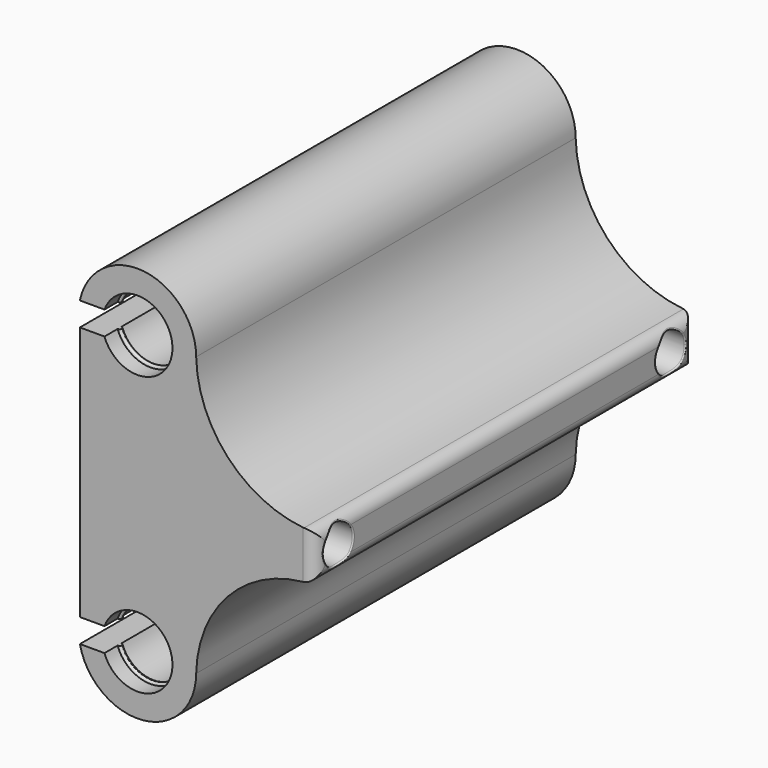
from build123d import *

# Parameters (mm, degrees)
F1_DEPTH      = 50.8
F2_R          = 4
F3_DEPTH      = 25.4
F4_T1_DEPTH   = 22.7
F4_T3_DEPTH   = 113.7216584723
F4_T5_DEPTH   = 113.721658441
F5_R          = 0.254
F8_DEPTH      = 0.9906
F11_T2_ANGLE  = 338.3178112703
F11_T4_ANGLE  = 338.3178112703
F11_T6_ANGLE  = 338.3178112703
F11_T8_ANGLE  = 338.3178112703
F11_T10_ANGLE = 338.3178112703
F11_T12_ANGLE = 338.3178112703
F11_T14_ANGLE = 338.3178112703
F11_T16_ANGLE = 338.3178112703


# Not quite as in the source:
# - a fillet or chamfer that OpenCascade refuses, or shapes differently, is made with other operations: its cross-section is extruded or revolved along the edge and cut away or added
# - ends of sketch curves that miss each other by under 0.0002 mm in the source are joined


with BuildPart() as f1:
    # F0 (on Front) → F1 (new body, symmetric)
    with BuildSketch(Plane.XZ):
        with BuildLine():
            ThreePointArc((-7.0574570763, 32.385), (7.50062, 29.845), (-7.0574570763, 27.305))
            Line((-7.0574570763, 27.305), (-12.3215420944, 27.305))
            Line((-12.3215420944, 27.305), (-12.3215420944, -27.305))
            Line((-12.3215420944, -27.305), (-7.0574570763, -27.305))
            ThreePointArc((-7.0574570763, -27.305), (7.50062, -29.845), (-7.0574570763, -32.385))
            Line((-7.0574570763, -32.385), (-12.3215420944, -32.385))
            ThreePointArc((-12.3215420944, -32.385), (1.2765893389, -42.3606829316), (12.58062, -29.845))
            ThreePointArc((12.58062, -29.845), (20.2152455374, -12.2439740194), (37.98062, -5))
            Line((37.98062, -5), (37.98062, 0))
            Line((37.98062, 0), (37.98062, 5))
            ThreePointArc((37.98062, 5), (20.2152461882, 12.2439733419), (12.58062, 29.845))
            ThreePointArc((12.58062, 29.845), (1.2765893389, 42.3606829316), (-12.3215420944, 32.385))
            Line((-12.3215420944, 32.385), (-7.0574570763, 32.385))
        make_face()
    extrude(amount=F1_DEPTH, both=True)

    # F2 (on face) → F3 (cut)
    with BuildSketch(Plane.YZ.offset(37.98062)):
        with Locations((-44.45, 0)):
            Circle(F2_R)
        with Locations((44.45, 0)):
            Circle(F2_R)
    extrude(amount=-F3_DEPTH, mode=Mode.SUBTRACT)

    # F4: fillet of radius 2.54 on 4 edges, made by hand

    # F4_s2 → F4_t1 (cut)
    with BuildSketch(Plane.XY.offset(-11.35)):
        with BuildLine():
            ThreePointArc((35.44062, -50.8), (37.2366712242, -50.0560512242), (37.98062, -48.26))
            Line((37.98062, -48.26), (37.98062, -50.8))
            Line((37.98062, -50.8), (35.44062, -50.8))
        make_face()
        with BuildLine():
            ThreePointArc((35.44062, 50.8), (37.2366712242, 50.0560512242), (37.98062, 48.26))
            Line((37.98062, 48.26), (37.98062, 50.8))
            Line((37.98062, 50.8), (35.44062, 50.8))
        make_face()
    extrude(amount=F4_T1_DEPTH, mode=Mode.SUBTRACT)

    # F4_s4 → F4_t3 (cut)
    with BuildSketch(Plane.XZ.offset(-56.8608292361)):
        with BuildLine():
            ThreePointArc((35.671477868, 5.1051553375), (37.3165169834, 4.2881549501), (37.98062, 2.5756683055))
            Line((37.98062, 2.5756683055), (37.98062, 5))
            ThreePointArc((37.98062, 5), (36.8248523945, 5.0263024486), (35.671477868, 5.1051553375))
        make_face()
    extrude(amount=F4_T3_DEPTH, mode=Mode.SUBTRACT)

    # F4_s6 → F4_t5 (cut)
    with BuildSketch(Plane.XZ.offset(-56.8608292205)):
        with BuildLine():
            ThreePointArc((35.6714778739, -5.1051553432), (37.3165169854, -4.2881549541), (37.98062, -2.5756683118))
            Line((37.98062, -2.5756683118), (37.98062, -5))
            ThreePointArc((37.98062, -5), (36.8248523974, -5.0263024516), (35.6714778739, -5.1051553432))
        make_face()
    extrude(amount=F4_T5_DEPTH, mode=Mode.SUBTRACT)

    # F5
    f5_edges = [f1.edges().sort_by_distance(p)[0] for p in [
        (37.543684, -44.45, 4),
        (37.98062, -47.951606, -1.933586),
        (37.98062, -40.69224, 1.370853),
        (37.98062, -47.951606, 1.933586),
        (37.98062, -40.69224, -1.370853),
        (37.973504, -48.45, 0),
        (37.543684, -44.45, -4),
        (37.543684, 44.45, 4),
        (37.97661, 48.402676, -0.613478),
        (37.97661, 48.402676, 0.613478),
        (37.543688, 44.44316, -3.999994),
        (37.98062, 47.951606, -1.933586),
        (37.98062, 47.951606, 1.933586),
        (37.98062, 40.45, 0),
    ]]
    fillet(f5_edges, radius=F5_R)

    # F7 (on offset) → F8 (join)
    with BuildSketch(Plane.XZ.offset(47.29988)):
        with BuildLine():
            ThreePointArc((-6.5149930518, 32.385), (6.99262, 29.845), (-6.5149930518, 27.305))
            Line((-6.5149930518, 27.305), (-7.0574570763, 27.305))
            ThreePointArc((-7.0574570763, 27.305), (7.50062, 29.845), (-7.0574570763, 32.385))
            Line((-7.0574570763, 32.385), (-6.5149930518, 32.385))
        make_face()
    extrude(amount=-F8_DEPTH)


with BuildPart() as f9_1:
    # F9: instance of F1
    add(f1.part.mirror(Plane.XY))


with BuildPart() as f1_1:
    add(f1.part)

    add(f9_1.part)  # F10 merges F9_1
    # F10: F9_1, F1 across plane
    add(f9_1.part.mirror(Plane.XZ))
    add(f1.part.mirror(Plane.XZ))

    # F11: fillet of radius 0.508 on 8 edges, made by hand

    # F11_s1 → F11_t2 (revolve, cut)
    with BuildSketch(Plane(origin=(5.5132355773, 0, 28.7891953424), x_dir=(0, 1, 0), z_dir=(-0.1880857941, 0, -0.9821526022))):
        with BuildLine():
            ThreePointArc((-47.29988, -13.1140405264), (-47.1510902448, -12.7548302815), (-46.79188, -12.6060405264))
            Line((-46.79188, -12.6060405264), (-47.29988, -12.6060405264))
            Line((-47.29988, -12.6060405264), (-47.29988, -13.1140405264))
        make_face()
    revolve(axis=Axis((0, -47.29988, 29.845), (0, 1, 0)), revolution_arc=F11_T2_ANGLE, mode=Mode.SUBTRACT)

    # F11_s3 → F11_t4 (revolve, cut)
    with BuildSketch(Plane(origin=(5.5132355773, 0, 28.7891953424), x_dir=(0, 1, 0), z_dir=(-0.1880857941, 0, -0.9821526022))):
        with BuildLine():
            ThreePointArc((-46.81728, -12.6060405264), (-46.4580697552, -12.7548302815), (-46.30928, -13.1140405264))
            Line((-46.30928, -13.1140405264), (-46.30928, -12.6060405264))
            Line((-46.30928, -12.6060405264), (-46.81728, -12.6060405264))
        make_face()
    revolve(axis=Axis((0, -46.30928, 29.845), (0, 1, 0)), revolution_arc=F11_T4_ANGLE, mode=Mode.SUBTRACT)

    # F11_s5 → F11_t6 (revolve, cut)
    with BuildSketch(Plane(origin=(5.5132355773, 0, 28.7891953424), x_dir=(0, 1, 0), z_dir=(-0.1880857941, 0, -0.9821526022))):
        with BuildLine():
            ThreePointArc((46.79188, -12.6060405264), (47.1510902448, -12.7548302815), (47.29988, -13.1140405264))
            Line((47.29988, -13.1140405264), (47.29988, -12.6060405264))
            Line((47.29988, -12.6060405264), (46.79188, -12.6060405264))
        make_face()
    revolve(axis=Axis((0, 47.29988, 29.845), (0, 1, 0)), revolution_arc=F11_T6_ANGLE, mode=Mode.SUBTRACT)

    # F11_s7 → F11_t8 (revolve, cut)
    with BuildSketch(Plane(origin=(5.5132355773, 0, 28.7891953424), x_dir=(0, 1, 0), z_dir=(-0.1880857941, 0, -0.9821526022))):
        with BuildLine():
            ThreePointArc((46.30928, -13.1140405264), (46.4580697552, -12.7548302815), (46.81728, -12.6060405264))
            Line((46.81728, -12.6060405264), (46.30928, -12.6060405264))
            Line((46.30928, -12.6060405264), (46.30928, -13.1140405264))
        make_face()
    revolve(axis=Axis((0, 46.30928, 29.845), (0, 1, 0)), revolution_arc=F11_T8_ANGLE, mode=Mode.SUBTRACT)

    # F11_s9 → F11_t10 (revolve, cut)
    with BuildSketch(Plane(origin=(5.5132355773, 0, -28.7891953424), x_dir=(0, 1, 0), z_dir=(-0.1880857941, 0, 0.9821526022))):
        with BuildLine():
            ThreePointArc((46.79188, 12.6060405264), (47.1510902448, 12.7548302815), (47.29988, 13.1140405264))
            Line((47.29988, 13.1140405264), (47.29988, 12.6060405264))
            Line((47.29988, 12.6060405264), (46.79188, 12.6060405264))
        make_face()
    revolve(axis=Axis((0, 47.29988, -29.845), (0, -1, 0)), revolution_arc=F11_T10_ANGLE, mode=Mode.SUBTRACT)

    # F11_s11 → F11_t12 (revolve, cut)
    with BuildSketch(Plane(origin=(5.5132355773, 0, -28.7891953424), x_dir=(0, 1, 0), z_dir=(-0.1880857941, 0, 0.9821526022))):
        with BuildLine():
            ThreePointArc((46.30928, 13.1140405264), (46.4580697552, 12.7548302815), (46.81728, 12.6060405264))
            Line((46.81728, 12.6060405264), (46.30928, 12.6060405264))
            Line((46.30928, 12.6060405264), (46.30928, 13.1140405264))
        make_face()
    revolve(axis=Axis((0, 46.30928, -29.845), (0, -1, 0)), revolution_arc=F11_T12_ANGLE, mode=Mode.SUBTRACT)

    # F11_s13 → F11_t14 (revolve, cut)
    with BuildSketch(Plane(origin=(5.5132355773, 0, -28.7891953424), x_dir=(0, 1, 0), z_dir=(-0.1880857941, 0, 0.9821526022))):
        with BuildLine():
            ThreePointArc((-46.81728, 12.6060405264), (-46.4580697552, 12.7548302815), (-46.30928, 13.1140405264))
            Line((-46.30928, 13.1140405264), (-46.30928, 12.6060405264))
            Line((-46.30928, 12.6060405264), (-46.81728, 12.6060405264))
        make_face()
    revolve(axis=Axis((0, -46.30928, -29.845), (0, -1, 0)), revolution_arc=F11_T14_ANGLE, mode=Mode.SUBTRACT)

    # F11_s15 → F11_t16 (revolve, cut)
    with BuildSketch(Plane(origin=(5.5132355773, 0, -28.7891953424), x_dir=(0, 1, 0), z_dir=(-0.1880857941, 0, 0.9821526022))):
        with BuildLine():
            ThreePointArc((-47.29988, 13.1140405264), (-47.1510902448, 12.7548302815), (-46.79188, 12.6060405264))
            Line((-46.79188, 12.6060405264), (-47.29988, 12.6060405264))
            Line((-47.29988, 12.6060405264), (-47.29988, 13.1140405264))
        make_face()
    revolve(axis=Axis((0, -47.29988, -29.845), (0, -1, 0)), revolution_arc=F11_T16_ANGLE, mode=Mode.SUBTRACT)


solid = f1_1.part
